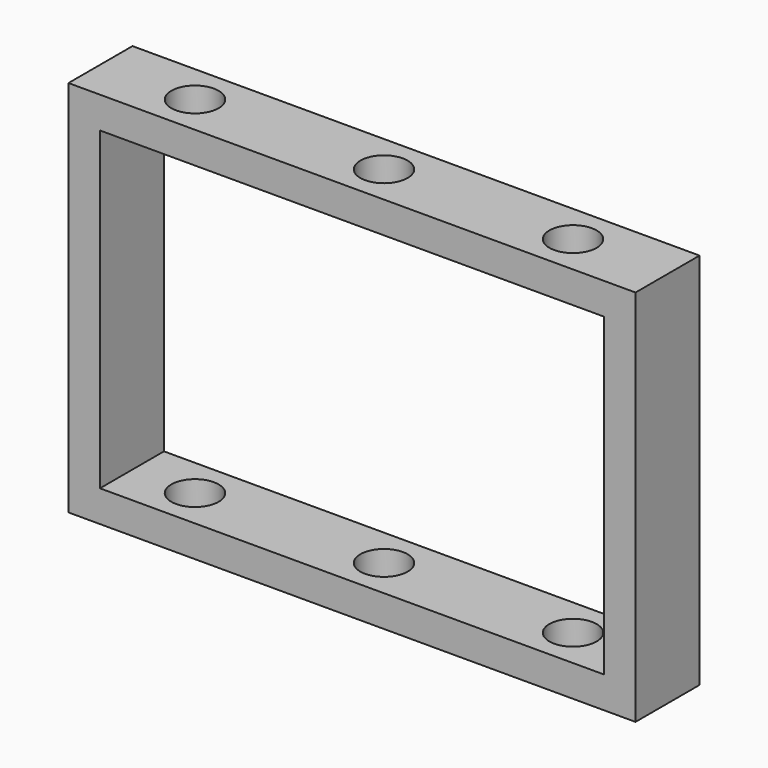
from build123d import *

# Parameters (mm, degrees)
F0_W     = 90
F0_H     = 60
F0_W_2   = 80
F0_H_2   = 50
F1_DEPTH = 12.7
F2_R     = 3.75
F3_DEPTH = 76.2


# Not quite as in the source:
# - a feature names something its author has since deleted; it is built from what else it names


with BuildPart() as f1:
    # F0 (on Front) → F1 (new body)
    with BuildSketch(Plane.XZ):
        Rectangle(F0_W, F0_H)
        Rectangle(F0_W_2, F0_H_2, mode=Mode.SUBTRACT)
    extrude(amount=F1_DEPTH)

    # F2 (on face) → F3 (cut)
    with BuildSketch(Plane(origin=(0, 0, -30), x_dir=(1, 0, 0), z_dir=(0, 0, -1))):
        with Locations((-30, 6.35)):
            Circle(F2_R)
        with Locations((0, 6.35)):
            Circle(F2_R)
        with Locations((30, 6.35)):
            Circle(F2_R)
    extrude(amount=-F3_DEPTH, mode=Mode.SUBTRACT)


solid = f1.part
